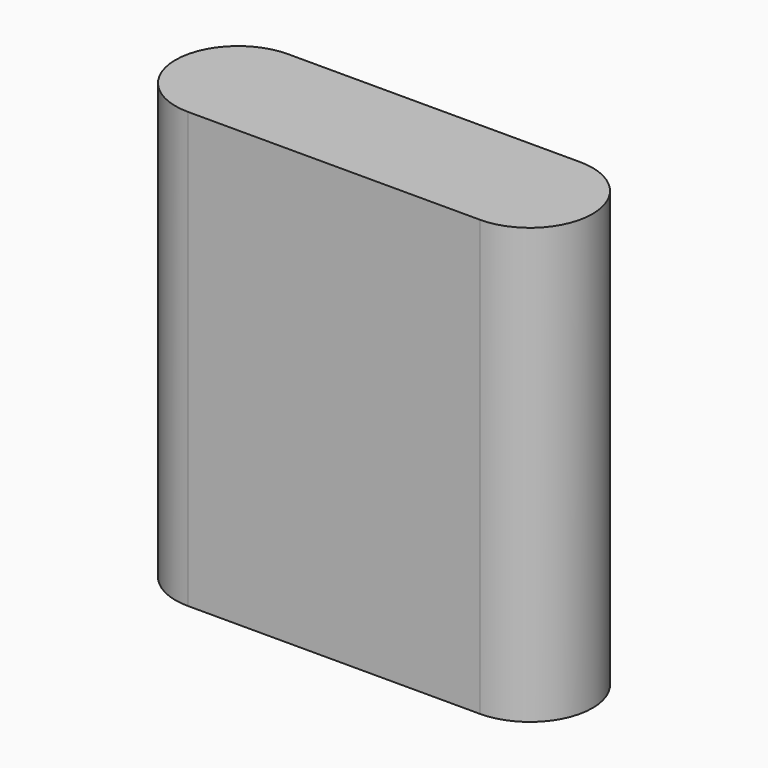
from build123d import *

# Parameters (mm, degrees)
F1_DEPTH = 25.4
F4_DEPTH = 40.8451128751


# Not quite as in the source:
# - the program builds the solid bodies; features that only make, move or delete a surface that nothing else refers to are left out


with BuildPart() as f1:
    # F0 (on Top) → F1 (new body)
    with BuildSketch(Plane.XY):
        with BuildLine():
            ThreePointArc((0, -9.525), (6.7351920908, -6.7351920908), (9.525, 0))
            ThreePointArc((9.525, 0), (6.7351920908, 6.7351920908), (0, 9.525))
            ThreePointArc((0, 9.525), (-9.525, 0), (0, -9.525))
        make_face()
        with BuildLine():
            ThreePointArc((0, 9.525), (6.7351920908, 6.7351920908), (9.525, 0))
            ThreePointArc((9.525, 0), (6.7351920908, -6.7351920908), (0, -9.525))
            Line((0, -9.525), (44.45, -9.525))
            ThreePointArc((44.45, -9.525), (34.925, 0), (44.45, 9.525))
            Line((44.45, 9.525), (0, 9.525))
        make_face()
        with BuildLine():
            ThreePointArc((53.975, 0), (51.1851920908, 6.7351920908), (44.45, 9.525))
            ThreePointArc((44.45, 9.525), (34.925, 0), (44.45, -9.525))
            ThreePointArc((44.45, -9.525), (51.1851920908, -6.7351920908), (53.975, 0))
        make_face()
    extrude(amount=F1_DEPTH)

    # F4 (add): a face of the model
    f4_faces = [f1.faces().sort_by_distance(p)[0] for p in [
        (22.225, 0, 0),
    ]]
    extrude(f4_faces, amount=F4_DEPTH)


solid = f1.part
